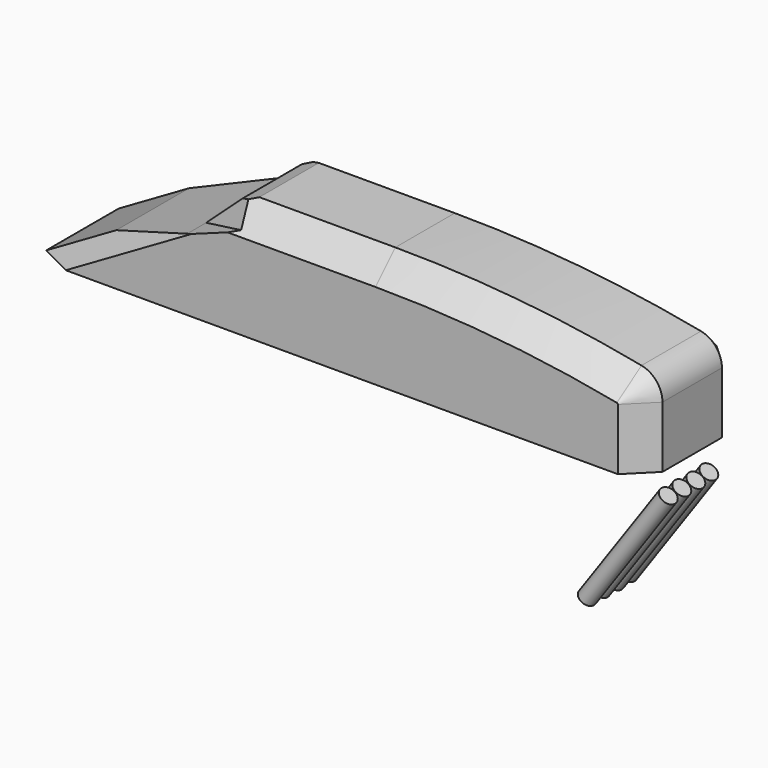
from build123d import *

# Parameters (mm, degrees)
F1_DEPTH     = 38.1
F2_T1_DEPTH  = 306.2724899177
F3_R         = 7.9805448281
F4_T1_DEPTH  = 54.3072830908
F4_T6_DEPTH  = 57.3260545127
F4_T11_DEPTH = 57.3260545127
F5_SIZE      = 5.08
F6_SIZE      = 7.62
F9_START     = 35.306
F8_R         = 2.54
F9_DEPTH     = 43.434
F10_R        = 2.241694022
F10_R_2      = 2.5705753266
F11_DEPTH    = 25.4


# Not quite as in the source:
# - a fillet or chamfer that OpenCascade refuses, or shapes differently, is made with other operations: its cross-section is extruded or revolved along the edge and cut away or added


with BuildPart() as f1:
    # F0 (on Front) → F1 (new body)
    with BuildSketch(Plane.XZ):
        Polygon((-117.0292248611, 12.5180522991), (-138.6344432831, 0), (-86.75300612, 0), (-54.147850991, 0), (0, 0), (48.9077347708, 0), (48.9077347708, 25.4), (20.3782214363, 34.0607471224), (0, 34.0607471224), (-28.8206309022, 34.0607471224), (-58.22349694, 34.0607471224), (-78.0194832408, 34.0607471224), (-91.4108872046, 21.8338113525), align=None)
    extrude(amount=F1_DEPTH)

    # F2: fillet of radius 394.0730054862 on 1 edges, made by hand

    # F2_s2 → F2_t1 (cut)
    with BuildSketch(Plane.XZ.offset(-134.0862449589)):
        with BuildLine():
            ThreePointArc((-33.2562765472, 34.0607471224), (8.0533267448, 31.8895792548), (48.9077347708, 25.4))
            Line((48.9077347708, 25.4), (20.3782214363, 34.0607471224))
            Line((20.3782214363, 34.0607471224), (-33.2562765472, 34.0607471224))
        make_face()
    extrude(amount=F2_T1_DEPTH, mode=Mode.SUBTRACT)

    # F3
    f3_edges = [f1.edges().sort_by_distance(p)[0] for p in [
        (48.907735, -19.05, 25.4),
    ]]
    fillet(f3_edges, radius=F3_R)

    # F4: chamfer of 7.62 on 3 edges, made by hand

    # F4_s2 → F4_t1 (cut)
    with BuildSketch(Plane.XZ.offset(-8.1036415454)):
        Polygon((-75.0640757299, 34.0607471224), (-80.2020086769, 32.0680062271), (-78.0194832408, 34.0607471224), align=None)
    extrude(amount=F4_T1_DEPTH, mode=Mode.SUBTRACT)


with BuildPart() as f4_tool4:
    # F4_s5 → F4_t6 (new body)
    with BuildSketch(Plane(origin=(-11.1170923555, 0, -10.1503900969), x_dir=(0, 1, 0), z_dir=(-0.7384854468, 0, -0.6742694156))):
        Polygon((-30.48, -77.7595174297), (-38.1, -70.1395174297), (-38.1, -77.7595174297), align=None)
    extrude(amount=F4_T6_DEPTH)

    split(bisect_by=Plane(origin=(-17.688042782, 0, 48.6421181436), x_dir=(0, 1, 0), z_dir=(-0.34174306, 0, 0.9397934246)), keep=Keep.TOP)


with BuildPart() as f1_1:
    add(f1.part)

    # F4_t3: cut F4_tool4
    add(f4_tool4.part, mode=Mode.SUBTRACT)


with BuildPart() as f4_tool9:
    # F4_s10 → F4_t11 (new body)
    with BuildSketch(Plane(origin=(-11.1170923555, 0, -10.1503900969), x_dir=(0, 1, 0), z_dir=(-0.7384854468, 0, -0.6742694156))):
        Polygon((0, -70.1395174297), (-7.62, -77.7595174297), (0, -77.7595174297), align=None)
    extrude(amount=F4_T11_DEPTH)

    split(bisect_by=Plane(origin=(-17.688042782, 0, 48.6421181436), x_dir=(0, 1, 0), z_dir=(-0.34174306, 0, 0.9397934246)), keep=Keep.TOP)


with BuildPart() as f1_2:
    add(f1_1.part)

    # F4_t8: cut F4_tool9
    add(f4_tool9.part, mode=Mode.SUBTRACT)

    # F5
    f5_edges = [f1_2.edges().sort_by_distance(p)[0] for p in [
        (-127.831834, -38.1, 6.259026),
        (-127.831834, 0, 6.259026),
    ]]
    chamfer(f5_edges, length=F5_SIZE)

    # F6
    f6_edges = [f1_2.edges().sort_by_distance(p)[0] for p in [
        (-49.98732, -38.1, 34.060747),
        (-49.98732, 0, 34.060747),
        (48.907735, 0, 9.443205),
        (4.779733, 0, 32.22083),
        (47.088613, 0, 23.958488),
        (48.907735, -38.1, 9.443205),
        (4.779733, -38.1, 32.22083),
        (47.088613, -38.1, 23.958488),
    ]]
    chamfer(f6_edges, length=F6_SIZE)

    # F10 (on Front) → F11 (cut)
    with BuildSketch(Plane.XZ):
        with Locations((-84.3102261424, 5.0523453392)):
            Circle(F10_R)
        with Locations((19.8654048145, 7.4005662464)):
            Circle(F10_R_2)
    extrude(amount=-F11_DEPTH, mode=Mode.SUBTRACT)


with BuildPart() as f9:
    # F8 (on face) → F9 (new body)
    with BuildSketch(Plane(origin=(26.5225739082, 0, 37.8781610607), x_dir=(0.8191520443, 0, -0.5735764364), z_dir=(-0.5735764364, 0, -0.8191520443)).offset(F9_START)):
        with Locations((41.1896929145, 1.5347069129)):
            Circle(F8_R)
    extrude(amount=F9_DEPTH)


with BuildPart() as f9b:
    # F8 (on face) → F9, piece 2 (new body)
    with BuildSketch(Plane(origin=(26.5225739082, 0, 37.8781610607), x_dir=(0.8191520443, 0, -0.5735764364), z_dir=(-0.5735764364, 0, -0.8191520443)).offset(F9_START)):
        with Locations((41.3663163781, 6.7077982239)):
            Circle(F8_R)
    extrude(amount=F9_DEPTH)


with BuildPart() as f9c:
    # F8 (on face) → F9, piece 3 (new body)
    with BuildSketch(Plane(origin=(26.5225739082, 0, 37.8781610607), x_dir=(0.8191520443, 0, -0.5735764364), z_dir=(-0.5735764364, 0, -0.8191520443)).offset(F9_START)):
        with Locations((41.259650141, 11.9897695258)):
            Circle(F8_R)
    extrude(amount=F9_DEPTH)


with BuildPart() as f9d:
    # F8 (on face) → F9, piece 4 (new body)
    with BuildSketch(Plane(origin=(26.5225739082, 0, 37.8781610607), x_dir=(0.8191520443, 0, -0.5735764364), z_dir=(-0.5735764364, 0, -0.8191520443)).offset(F9_START)):
        with Locations((41.2946268916, 17.2172989696)):
            Circle(F8_R)
    extrude(amount=F9_DEPTH)


solid = Compound([f1_2.part, f9.part, f9b.part, f9c.part, f9d.part])
